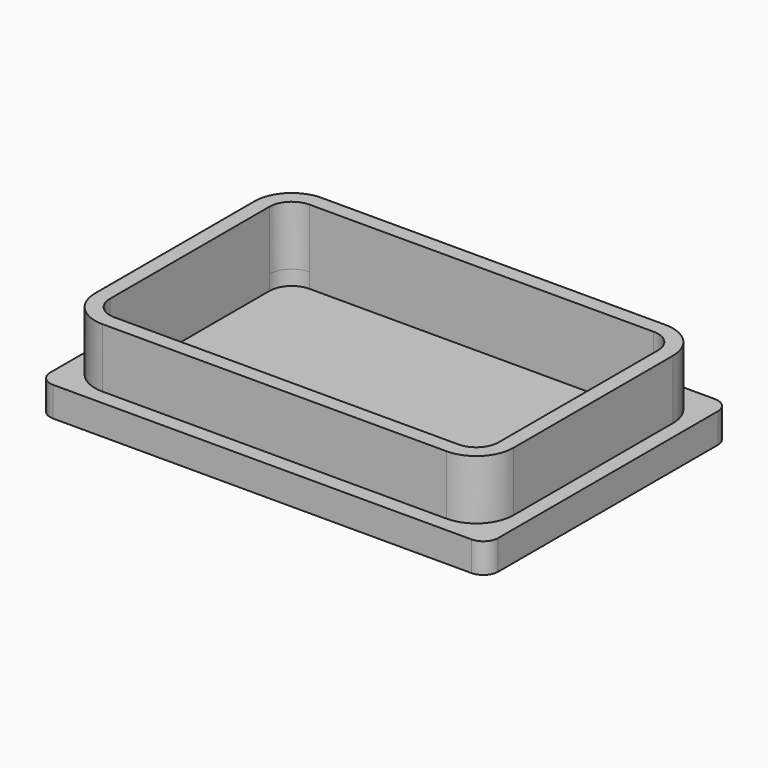
from build123d import *

# Parameters (mm, degrees)
F1_DEPTH     = 5.08
F3_DEPTH     = 15.24
F4_T         = 2.54
F4_T3_DEPTH  = 64.008
F4_T5_DEPTH  = 39.243
F4_T8_ANGLE  = 90.000000001
F4_T10_ANGLE = 90.000000001
F4_T12_ANGLE = 90.000000001
F4_T14_ANGLE = 90.000000001


# Not quite as in the source:
# - a shell that OpenCascade refuses in one call is made with other operations: the cavity is built on its own and cut out
# - the program builds the solid bodies; features that only make, move or delete a surface that nothing else refers to are left out


with BuildPart() as f1:
    # F0 (on Top) → F1 (new body)
    with BuildSketch(Plane.XY):
        with BuildLine():
            Line((35.814, 26.035), (-35.814, 26.035))
            ThreePointArc((-35.814, 26.035), (-37.6100512242, 25.2910512242), (-38.354, 23.495))
            Line((-38.354, 23.495), (-38.354, -23.495))
            ThreePointArc((-38.354, -23.495), (-37.6100512242, -25.2910512242), (-35.814, -26.035))
            Line((-35.814, -26.035), (35.814, -26.035))
            ThreePointArc((35.814, -26.035), (37.6100512242, -25.2910512242), (38.354, -23.495))
            Line((38.354, -23.495), (38.354, 23.495))
            ThreePointArc((38.354, 23.495), (37.6100512242, 25.2910512242), (35.814, 26.035))
        make_face()
        with BuildLine():
            ThreePointArc((-35.814, 17.0815), (-33.9541280605, 21.5716280605), (-29.464, 23.4315))
            Line((-29.464, 23.4315), (29.464, 23.4315))
            ThreePointArc((29.464, 23.4315), (33.9541280605, 21.5716280605), (35.814, 17.0815))
            Line((35.814, 17.0815), (35.814, -17.0815))
            ThreePointArc((35.814, -17.0815), (33.9541280605, -21.5716280605), (29.464, -23.4315))
            Line((29.464, -23.4315), (-29.464, -23.4315))
            ThreePointArc((-29.464, -23.4315), (-33.9541280605, -21.5716280605), (-35.814, -17.0815))
            Line((-35.814, -17.0815), (-35.814, 17.0815))
        make_face(mode=Mode.SUBTRACT)
    extrude(amount=F1_DEPTH)

    # F0 (on Top) → F3 (join)
    with BuildSketch(Plane.XY):
        with BuildLine():
            Line((29.464, 23.4315), (-29.464, 23.4315))
            ThreePointArc((-29.464, 23.4315), (-33.9541280605, 21.5716280605), (-35.814, 17.0815))
            Line((-35.814, 17.0815), (-35.814, -17.0815))
            ThreePointArc((-35.814, -17.0815), (-33.9541280605, -21.5716280605), (-29.464, -23.4315))
            Line((-29.464, -23.4315), (29.464, -23.4315))
            ThreePointArc((29.464, -23.4315), (33.9541280605, -21.5716280605), (35.814, -17.0815))
            Line((35.814, -17.0815), (35.814, 17.0815))
            ThreePointArc((35.814, 17.0815), (33.9541280605, 21.5716280605), (29.464, 23.4315))
        make_face()
    extrude(amount=F3_DEPTH)

    # F4: shell of thickness 2.54, made by hand


with BuildPart() as f4_core1:
    # F4_t2: copy of F1
    add(f1.part)

    # the walls: a layer under each face that stays
    f4_faces = [f4_core1.faces().sort_by_distance(p)[0] for p in [
        (0, 26.035, 2.54),
        (0, 0, 0),
        (-35.7970666667, -24.2993333333, 5.08),
        (38.354, 0, 2.54),
        (-38.354, 0, 2.54),
        (0, -26.035, 2.54),
        (-33.9541280605, 21.5716280605, 10.16),
        (0, 23.4315, 10.16),
        (33.9541280605, 21.5716280605, 10.16),
        (35.814, 0, 10.16),
        (33.9541280605, -21.5716280605, 10.16),
        (0, -23.4315, 10.16),
        (-33.9541280605, -21.5716280605, 10.16),
        (-35.814, 0, 10.16),
    ]]
    thicken(f4_faces, amount=-F4_T, mode=Mode.SUBTRACT)

    # F4_s4 → F4_t3 (cut)
    with BuildSketch(Plane.YZ.offset(-32.004)):
        Polygon((23.4569, 5.1054), (23.4315, 2.54), (20.8915, 2.54), (20.8915, 5.08), align=None)
        Polygon((-23.4569, 5.1054), (-23.4315, 2.54), (-20.8915, 2.54), (-20.8915, 5.08), align=None)
    extrude(amount=F4_T3_DEPTH, mode=Mode.SUBTRACT)

    # F4_s6 → F4_t5 (cut)
    with BuildSketch(Plane.XZ.offset(-19.6215)):
        Polygon((35.8394, 5.1054), (35.814, 2.54), (33.274, 2.54), (33.274, 5.08), align=None)
        Polygon((-35.8394, 5.1054), (-35.814, 2.54), (-33.274, 2.54), (-33.274, 5.08), align=None)
    extrude(amount=F4_T5_DEPTH, mode=Mode.SUBTRACT)

    # F4_s7 → F4_t8 (revolve, cut)
    with BuildSketch(Plane.XZ.offset(-17.0815)):
        Polygon((-35.8394, 5.1054), (-35.814, 2.54), (-33.274, 2.54), (-33.274, 5.08), align=None)
    revolve(axis=Axis((-29.464, 17.0815, 5.08), (0, 0, -1)), revolution_arc=F4_T8_ANGLE, mode=Mode.SUBTRACT)

    # F4_s9 → F4_t10 (revolve, cut)
    with BuildSketch(Plane.YZ.offset(29.464)):
        Polygon((23.4569, 5.1054), (23.4315, 2.54), (20.8915, 2.54), (20.8915, 5.08), align=None)
    revolve(axis=Axis((29.464, 17.0815, 5.08), (0, 0, -1)), revolution_arc=F4_T10_ANGLE, mode=Mode.SUBTRACT)

    # F4_s11 → F4_t12 (revolve, cut)
    with BuildSketch(Plane.XZ.offset(17.0815)):
        Polygon((35.8394, 5.1054), (35.814, 2.54), (33.274, 2.54), (33.274, 5.08), align=None)
    revolve(axis=Axis((29.464, -17.0815, 5.08), (0, 0, -1)), revolution_arc=F4_T12_ANGLE, mode=Mode.SUBTRACT)

    # F4_s13 → F4_t14 (revolve, cut)
    with BuildSketch(Plane.YZ.offset(-29.464)):
        Polygon((-23.4569, 5.1054), (-23.4315, 2.54), (-20.8915, 2.54), (-20.8915, 5.08), align=None)
    revolve(axis=Axis((-29.464, -17.0815, 5.08), (0, 0, -1)), revolution_arc=F4_T14_ANGLE, mode=Mode.SUBTRACT)


with BuildPart() as f1_1:
    add(f1.part)

    # what is left inside the walls is the cavity
    f4_cavity = [f4_core1.part.solids().sort_by_distance(p)[0] for p in [
        (0, -6.963833, 2.5654),
    ]]
    add(f4_cavity, mode=Mode.SUBTRACT)


solid = f1_1.part
